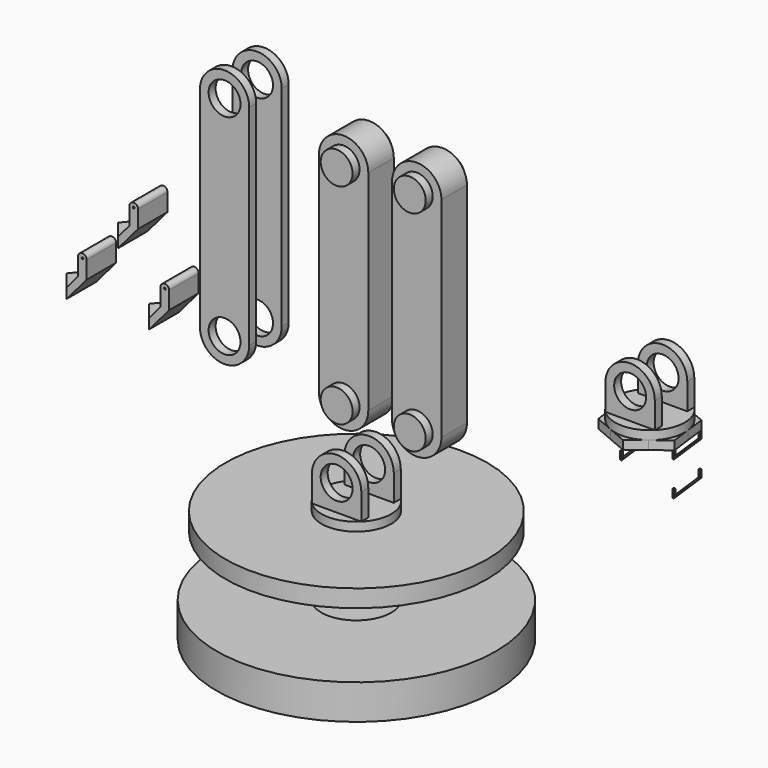
from build123d import *

# Parameters (mm, degrees)
F0_W      = 12.7
F0_H      = 3.175
F2_W      = 17.9605122421
F2_H      = 17.9605122421
F3_DEPTH  = 3.175
F4_W      = 17.9605122421
F4_H      = 3.175
F5_DEPTH  = 6.35
F7_DEPTH  = 3.175
F8_DEPTH  = 25.4
F10_DEPTH = 3.175
F11_DEPTH = 3.175
F13_DEPTH = 5.8039
F14_DEPTH = 8.9789
F17_DEPTH = 8.9789
F18_W     = 11.6078
F18_H     = 20.9132400393
F18_H_2   = 76.2
F19_DEPTH = 25.4
F21_DEPTH = 6.35
F23_DEPTH = 3.175
F25_DEPTH = 0.635
F26_R     = 0.31749
F29_W     = 5.4027563135
F29_H     = 3.7201785082
F30_DEPTH = 6.6929
F32_DEPTH = 25.4


# Not quite as in the source:
# - a fillet or chamfer is up to 0.001 mm smaller than in the source, because OpenCascade refuses the exact size


with BuildPart() as f1:
    # F0 (on Front) → F1 (revolve)
    with BuildSketch(Plane.XZ):
        Polygon((0, -73.4391258749), (0, -76.6141258749), (50.8, -76.6141258749), (50.8, -63.9141258749), (12.7, -63.9141258749), (12.7, -67.0891258749), (47.625, -67.0891258749), (47.625, -73.4391258749), align=None)
    revolve(axis=Axis((0, 0, 1.2423854659), (0, 0, 1)))


with BuildPart() as f1b:
    # F0 (on Front) → F1, piece 2 (revolve)
    with BuildSketch(Plane.XZ):
        Polygon((0, -35.4759466345), (0, -41.8259466345), (47.625, -41.8259466345), (47.625, -35.4759466345), (12.7, -35.4759466345), align=None)
        with Locations((6.35, -33.8884466345)):
            Rectangle(F0_W, F0_H)
    revolve(axis=Axis((0, 0, 1.2423854659), (0, 0, 1)))

    # F2 (on face) → F3 (join)
    with BuildSketch(Plane.XY.offset(-32.3009466345)):
        Rectangle(F2_W, F2_H)
    extrude(amount=F3_DEPTH)

    # F4 (on face) → F5 (join)
    with BuildSketch(Plane.XY.offset(-29.1259466345)):
        with Locations((0, 7.3927561211)):
            Rectangle(F4_W, F4_H)
        with Locations((0, -7.3927561211)):
            Rectangle(F4_W, F4_H)
    extrude(amount=F5_DEPTH)

    # F6 (on face) → F7 (join)
    with BuildSketch(Plane(origin=(0, 8.9802561211, 0), x_dir=(-1, 0, 0), z_dir=(0, 1, 0))):
        with BuildLine():
            Line((5.8052561211, -22.7759466345), (8.9802561211, -22.7759466345))
            ThreePointArc((8.9802561211, -22.7759466345), (0, -13.7956905134), (-8.9802561211, -22.7759466345))
            Line((-8.9802561211, -22.7759466345), (-5.8052561211, -22.7759466345))
            ThreePointArc((-5.8052561211, -22.7759466345), (0, -16.9706905134), (5.8052561211, -22.7759466345))
        make_face()
    extrude(amount=-F7_DEPTH)

    # F6 (on face) → F8 (cut)
    with BuildSketch(Plane(origin=(0, 8.9802561211, 0), x_dir=(-1, 0, 0), z_dir=(0, 1, 0))):
        with BuildLine():
            ThreePointArc((-5.8052561211, -22.7759466345), (0, -28.5812027556), (5.8052561211, -22.7759466345))
            Line((5.8052561211, -22.7759466345), (-5.8052561211, -22.7759466345))
        make_face()
        with BuildLine():
            Line((-5.8052561211, -22.7759466345), (5.8052561211, -22.7759466345))
            ThreePointArc((5.8052561211, -22.7759466345), (0, -16.9706905134), (-5.8052561211, -22.7759466345))
        make_face()
    extrude(amount=-F8_DEPTH, mode=Mode.SUBTRACT)

    # F9 (on face) → F10 (join)
    with BuildSketch(Plane.XZ.offset(8.9802561211)):
        with BuildLine():
            Line((5.8052561211, -22.7759466345), (8.9802561211, -22.7759466345))
            ThreePointArc((8.9802561211, -22.7759466345), (0, -13.7956905134), (-8.9802561211, -22.7759466345))
            Line((-8.9802561211, -22.7759466345), (-5.8052561211, -22.7759466345))
            ThreePointArc((-5.8052561211, -22.7759466345), (0, -16.9706905134), (5.8052561211, -22.7759466345))
        make_face()
    extrude(amount=-F10_DEPTH)

    # F11 (cut): a face of the model
    f11_faces = [f1b.faces().sort_by_distance(p)[0] for p in [
        (0, 0, -29.1259466345),
    ]]
    extrude(f11_faces, amount=-F11_DEPTH, mode=Mode.SUBTRACT)


with BuildPart() as f13:
    # F12 (on Front) → F13 (new body, symmetric)
    with BuildSketch(Plane.XZ):
        with BuildLine():
            Line((8.9789, 1.9930543381), (8.9789, 78.1930543381))
            Line((8.9789, 78.1930543381), (5.8039, 78.1930543381))
            ThreePointArc((5.8039, 78.1930543381), (0, 72.3891543381), (-5.8039, 78.1930543381))
            Line((-5.8039, 78.1930543381), (-8.9789, 78.1930543381))
            Line((-8.9789, 78.1930543381), (-8.9789, 1.9930543381))
            Line((-8.9789, 1.9930543381), (-5.8039, 1.9930543381))
            ThreePointArc((-5.8039, 1.9930543381), (0, 7.7969543381), (5.8039, 1.9930543381))
            Line((5.8039, 1.9930543381), (8.9789, 1.9930543381))
        make_face()
        with BuildLine():
            Line((5.8039, 78.1930543381), (8.9789, 78.1930543381))
            ThreePointArc((8.9789, 78.1930543381), (0, 87.1719543381), (-8.9789, 78.1930543381))
            Line((-8.9789, 78.1930543381), (-5.8039, 78.1930543381))
            ThreePointArc((-5.8039, 78.1930543381), (0, 83.9969543381), (5.8039, 78.1930543381))
        make_face()
        with BuildLine():
            ThreePointArc((-8.9789, 1.9930543381), (0, -6.9858456619), (8.9789, 1.9930543381))
            Line((8.9789, 1.9930543381), (5.8039, 1.9930543381))
            ThreePointArc((5.8039, 1.9930543381), (0, -3.8108456619), (-5.8039, 1.9930543381))
            Line((-5.8039, 1.9930543381), (-8.9789, 1.9930543381))
        make_face()
    extrude(amount=F13_DEPTH, both=True)

    # F12 (on Front) → F14 (join, symmetric)
    with BuildSketch(Plane.XZ):
        with BuildLine():
            Line((-5.8039, 1.9930543381), (5.8039, 1.9930543381))
            ThreePointArc((5.8039, 1.9930543381), (0, 7.7969543381), (-5.8039, 1.9930543381))
        make_face()
        with BuildLine():
            ThreePointArc((-5.8039, 1.9930543381), (0, -3.8108456619), (5.8039, 1.9930543381))
            Line((5.8039, 1.9930543381), (-5.8039, 1.9930543381))
        make_face()
        with BuildLine():
            ThreePointArc((-5.8039, 78.1930543381), (0, 72.3891543381), (5.8039, 78.1930543381))
            Line((5.8039, 78.1930543381), (-5.8039, 78.1930543381))
        make_face()
        with BuildLine():
            Line((-5.8039, 78.1930543381), (5.8039, 78.1930543381))
            ThreePointArc((5.8039, 78.1930543381), (0, 83.9969543381), (-5.8039, 78.1930543381))
        make_face()
    extrude(amount=F14_DEPTH, both=True)


with BuildPart() as f15_1:
    # F15: copy of F13
    add(f13.part.moved(Location((26.61451, 0, 0))))


with BuildPart() as f17:
    # F16 (on Front) → F17 (new body, symmetric)
    with BuildSketch(Plane.XZ):
        with BuildLine():
            Line((-31.8052559499, 10.945689404), (-31.8052559499, 87.145689404))
            Line((-31.8052559499, 87.145689404), (-34.9802559499, 87.145689404))
            ThreePointArc((-34.9802559499, 87.145689404), (-40.7841559499, 81.341789404), (-46.5880559499, 87.145689404))
            Line((-46.5880559499, 87.145689404), (-49.7630559499, 87.145689404))
            Line((-49.7630559499, 87.145689404), (-49.7630559499, 10.945689404))
            Line((-49.7630559499, 10.945689404), (-46.5880559499, 10.945689404))
            ThreePointArc((-46.5880559499, 10.945689404), (-40.7841559499, 16.749589404), (-34.9802559499, 10.945689404))
            Line((-34.9802559499, 10.945689404), (-31.8052559499, 10.945689404))
        make_face()
        with BuildLine():
            ThreePointArc((-49.7630559499, 10.945689404), (-40.7841559499, 1.966789404), (-31.8052559499, 10.945689404))
            Line((-31.8052559499, 10.945689404), (-34.9802559499, 10.945689404))
            ThreePointArc((-34.9802559499, 10.945689404), (-40.7841559499, 5.141789404), (-46.5880559499, 10.945689404))
            Line((-46.5880559499, 10.945689404), (-49.7630559499, 10.945689404))
        make_face()
        with BuildLine():
            Line((-34.9802559499, 87.145689404), (-31.8052559499, 87.145689404))
            ThreePointArc((-31.8052559499, 87.145689404), (-40.7841559499, 96.124589404), (-49.7630559499, 87.145689404))
            Line((-49.7630559499, 87.145689404), (-46.5880559499, 87.145689404))
            ThreePointArc((-46.5880559499, 87.145689404), (-40.7841559499, 92.949589404), (-34.9802559499, 87.145689404))
        make_face()
    extrude(amount=F17_DEPTH, both=True)

    # F18 (on face) → F19 (cut)
    with BuildSketch(Plane.YZ.offset(-31.8052559499)):
        with Locations((0, 97.6023094237)):
            Rectangle(F18_W, F18_H)
        with Locations((0, 49.045689404)):
            Rectangle(F18_W, F18_H_2)
        with Locations((0, 0.4890693843)):
            Rectangle(F18_W, F18_H)
    extrude(amount=-F19_DEPTH, mode=Mode.SUBTRACT)


with BuildPart() as f20_1:
    # F20: copy of F1b
    add(f1b.part.moved(Location((106.81246, 0, 64.0534))))

    # F21 (cut): a face of the model
    f21_faces = [f20_1.faces().sort_by_distance(p)[0] for p in [
        (106.81246, 0, 22.2274533655),
    ]]
    extrude(f21_faces, amount=-F21_DEPTH, mode=Mode.SUBTRACT)

    # F22 (on face) → F23 (join)
    with BuildSketch(Plane(origin=(0, 0, 28.5774533655), x_dir=(1, 0, 0), z_dir=(0, 0, -1))):
        with BuildLine():
            Line((118.5134517826, -8.8396903021), (119.415902043, -1.5630894631))
            ThreePointArc((119.415902043, -1.5630894631), (116.9458161788, -7.6553963029), (111.7605056119, -11.6964458115))
            Line((111.7605056119, -11.6964458115), (118.5134517826, -8.8396903021))
        make_face()
        with BuildLine():
            Line((105.007559528, -14.5532012842), (111.7605056119, -11.6964458115))
            ThreePointArc((111.7605056119, -11.6964458115), (105.2493701921, -12.6034420002), (99.1570634365, -10.1333559819))
            Line((99.1570634365, -10.1333559819), (105.007559528, -14.5532012842))
        make_face()
        with BuildLine():
            ThreePointArc((99.1570634365, -10.1333559819), (95.1160141966, -4.9480456311), (94.209017957, 1.5630894631))
            Line((94.209017957, 1.5630894631), (93.3065677455, -5.7135109821))
            Line((93.3065677455, -5.7135109821), (99.1570634365, -10.1333559819))
        make_face()
        with BuildLine():
            ThreePointArc((94.209017957, 1.5630894631), (96.6791037652, 7.6553962287), (101.8644142168, 11.6964457391))
            Line((101.8644142168, 11.6964457391), (95.1114682174, 8.8396903021))
            Line((95.1114682174, 8.8396903021), (94.209017957, 1.5630894631))
        make_face()
        with BuildLine():
            ThreePointArc((101.8644142168, 11.6964457391), (108.3755495971, 12.6034420263), (114.4678563728, 10.1333561259))
            Line((114.4678563728, 10.1333561259), (108.617360472, 14.5532012842))
            Line((108.617360472, 14.5532012842), (101.8644142168, 11.6964457391))
        make_face()
        with BuildLine():
            ThreePointArc((114.4678563728, 10.1333561259), (118.1815746079, 5.6597909001), (119.51246, 0))
            ThreePointArc((119.51246, 0), (119.4882975255, -0.7830344994), (119.415902043, -1.5630894631))
            Line((119.415902043, -1.5630894631), (120.3183522545, 5.7135109821))
            Line((120.3183522545, 5.7135109821), (114.4678563728, 10.1333561259))
        make_face()
        with BuildLine():
            ThreePointArc((119.415902043, -1.5630894631), (119.4882975255, -0.7830344994), (119.51246, 0))
            ThreePointArc((119.51246, 0), (118.1815746079, 5.6597909001), (114.4678563728, 10.1333561259))
            ThreePointArc((114.4678563728, 10.1333561259), (108.3755495971, 12.6034420263), (101.8644142168, 11.6964457391))
            ThreePointArc((101.8644142168, 11.6964457391), (96.6791037652, 7.6553962287), (94.209017957, 1.5630894631))
            ThreePointArc((94.209017957, 1.5630894631), (95.1160141966, -4.9480456311), (99.1570634365, -10.1333559819))
            ThreePointArc((99.1570634365, -10.1333559819), (105.2493701921, -12.6034420002), (111.7605056119, -11.6964458115))
            ThreePointArc((111.7605056119, -11.6964458115), (116.9458161788, -7.6553963029), (119.415902043, -1.5630894631))
        make_face()
    extrude(amount=F23_DEPTH)


with BuildPart() as f25:
    # F24 (on face) → F25 (new body)
    with BuildSketch(Plane(origin=(117.7978880899, 14.6093948442, 0), x_dir=(-0.123077926, 0.9923970093, 0), z_dir=(0.9923970093, 0.123077926, 0))):
        Polygon((-19.8436044649, 25.4024533655), (-20.4786044649, 25.4024533655), (-20.4786044649, 22.4047936499), (-5.8139076275, 22.4047936499), (-5.8139076275, 25.4024533655), (-6.4489076275, 25.4024533655), (-6.4489076275, 23.0397936499), (-19.8436044649, 23.0397936499), align=None)
    extrude(amount=-F25_DEPTH)

    # F26 (radius 0.3175 in the source; OpenCascade refuses exactly that, so slightly less here)
    f26_edges = [f25.edges().sort_by_distance(p)[0] for p in [
        (119.415902, 1.56309, 22.404794),
        (118.78573, 1.484935, 23.039794),
        (119.415902, 1.56309, 23.039794),
        (118.78573, 1.484935, 22.404794),
    ]]
    fillet(f26_edges, radius=F26_R)


with BuildPart() as f27_1:
    # F27: copy of F25
    add(f25.part.moved(Location((-19.05719, 0, -6.49677))))


with BuildPart() as f28_1:
    # F28: copy of F25
    add(f25.part.moved(Location((0, 0, -12.4738))))


with BuildPart() as f30:
    # F29 (on Front) → F30 (new body, symmetric)
    with BuildSketch(Plane.XZ):
        with BuildLine():
            Line((-92.7707294504, 17.5563662089), (-94.0280294504, 17.5563662089))
            ThreePointArc((-94.0280294504, 17.5563662089), (-94.3582294504, 17.2261662089), (-94.6884294504, 17.5563662089))
            Line((-94.6884294504, 17.5563662089), (-95.9457294504, 17.5563662089))
            Line((-95.9457294504, 17.5563662089), (-95.9457294504, 11.2063662089))
            Line((-95.9457294504, 11.2063662089), (-92.7707294504, 11.2063662089))
            Line((-92.7707294504, 11.2063662089), (-92.7707294504, 17.5563662089))
        make_face()
        with BuildLine():
            ThreePointArc((-94.6884294504, 17.5563662089), (-94.3582294504, 17.8865662089), (-94.0280294504, 17.5563662089))
            Line((-94.0280294504, 17.5563662089), (-92.7707294504, 17.5563662089))
            ThreePointArc((-92.7707294504, 17.5563662089), (-94.3582294504, 19.1438662089), (-95.9457294504, 17.5563662089))
            Line((-95.9457294504, 17.5563662089), (-94.6884294504, 17.5563662089))
        make_face()
        Polygon((-100.0679731369, 2.656114514), (-92.7707294504, 11.2063662089), (-95.9457294504, 11.2063662089), (-100.0679731369, 6.3762930222), align=None)
        with Locations((-102.7693512937, 4.5162037681)):
            Rectangle(F29_W, F29_H)
    extrude(amount=F30_DEPTH, both=True)

    # F31 (on face) → F32 (cut)
    with BuildSketch(Plane.XY.offset(6.3762930222)):
        Polygon((-105.4707294504, -6.6929), (-100.0679731369, -6.6929), (-105.4707294504, 0), align=None)
        Polygon((-105.4707294504, 6.6929), (-105.4707294504, 0), (-100.0679731369, 6.6929), align=None)
    extrude(amount=-F32_DEPTH, mode=Mode.SUBTRACT)


with BuildPart() as f33_1:
    # F33: copy of F30
    add(f30.part.moved(Location((30.01697, 0, 0))))


with BuildPart() as f34_1:
    # F34: copy of F30
    add(f30.part.moved(Location((18.68761, 0, 22.30833))))


solid = Compound([f1.part, f1b.part, f13.part, f15_1.part, f17.part, f20_1.part, f25.part, f27_1.part, f28_1.part, f30.part, f33_1.part, f34_1.part])
